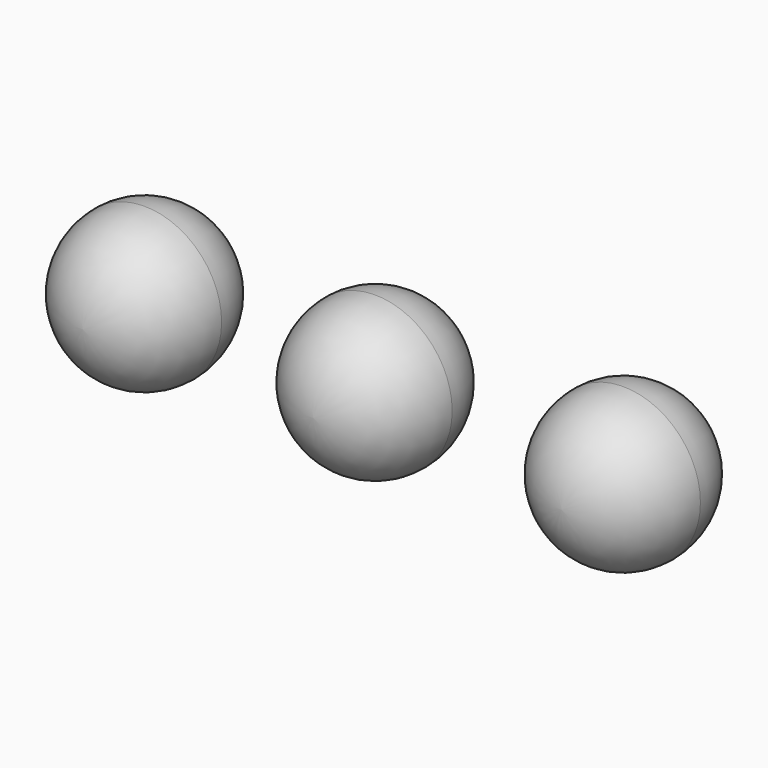
from build123d import *

# Parameters (mm, degrees)
F0_R     = 12.7
F1_DEPTH = 25.4
F2_R     = 12.69999
F3_R     = 12.69999
F4_R     = 12.69999


# Not quite as in the source:
# - a fillet or chamfer is up to 0.001 mm smaller than in the source, because OpenCascade refuses the exact size


with BuildPart() as f1:
    # F0 (on Front) → F1 (new body)
    with BuildSketch(Plane.XZ):
        Circle(F0_R)
    extrude(amount=F1_DEPTH)

    # F2 (radius 12.7 in the source; OpenCascade refuses exactly that, so slightly less here)
    f2_edges = [f1.edges().sort_by_distance(p)[0] for p in [
        (-12.7, 0, 0),
        (-12.7, -25.4, 0),
    ]]
    fillet(f2_edges, radius=F2_R)


with BuildPart() as f1b:
    # F0 (on Front) → F1, piece 2 (new body)
    with BuildSketch(Plane.XZ):
        with Locations((-37.9858093821, 0.5063325813)):
            Circle(F0_R)
    extrude(amount=F1_DEPTH)

    # F3 (radius 12.7 in the source; OpenCascade refuses exactly that, so slightly less here)
    f3_edges = [f1b.edges().sort_by_distance(p)[0] for p in [
        (-50.685809, -25.4, 0.506333),
        (-50.685809, 0, 0.506333),
    ]]
    fillet(f3_edges, radius=F3_R)


with BuildPart() as f1c:
    # F0 (on Front) → F1, piece 3 (new body)
    with BuildSketch(Plane.XZ):
        with Locations((40.8935248852, 0)):
            Circle(F0_R)
    extrude(amount=F1_DEPTH)

    # F4 (radius 12.7 in the source; OpenCascade refuses exactly that, so slightly less here)
    f4_edges = [f1c.edges().sort_by_distance(p)[0] for p in [
        (28.193525, -25.4, 0),
        (28.193525, 0, 0),
    ]]
    fillet(f4_edges, radius=F4_R)


solid = Compound([f1.part, f1b.part, f1c.part])
